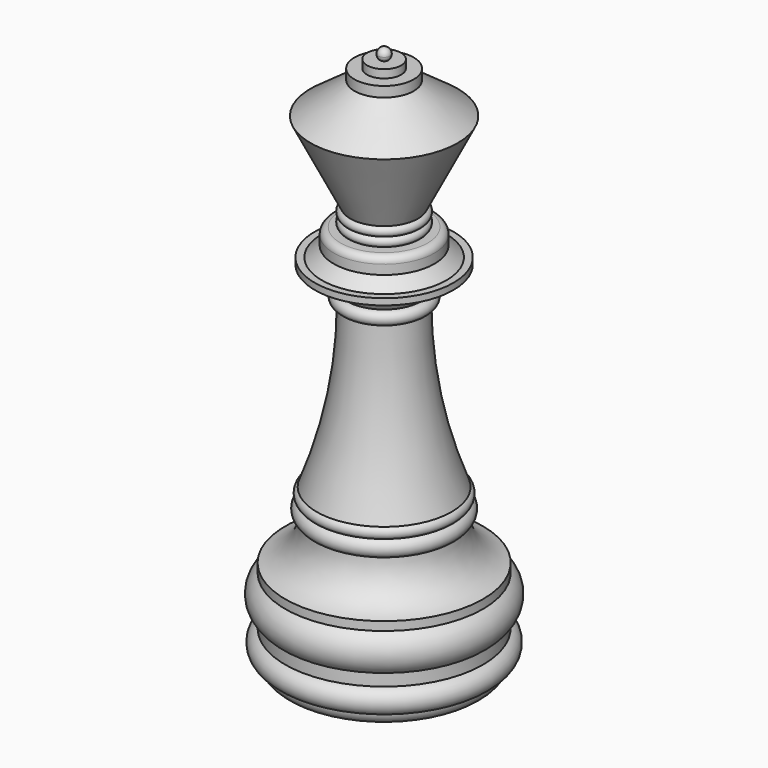
from build123d import *

# Parameters (mm, degrees)
F6_R     = 1
F8_R     = 0.896765
F9_DEPTH = 1.79353
F10_R    = 0.896755


# Not quite as in the source:
# - a fillet or chamfer that OpenCascade refuses, or shapes differently, is made with other operations: its cross-section is extruded or revolved along the edge and cut away or added
# - a fillet or chamfer is up to 0.001 mm smaller than in the source, because OpenCascade refuses the exact size


with BuildPart() as f1:
    # F0 (on Front) → F1 (revolve)
    with BuildSketch(Plane.XZ):
        with BuildLine():
            Line((-200.8288223515, 101.2477203459), (-203.3652514219, 101.2477203459))
            Line((-203.3652514219, 101.2477203459), (-203.3652514219, 21.2477203459))
            Line((-203.3652514219, 21.2477203459), (-188.6436624619, 21.2477203459))
            Line((-188.6436624619, 21.2477203459), (-188.6436624619, 23.0397097766))
            ThreePointArc((-188.6436624619, 23.0397097766), (-187.333962533, 24.8457370326), (-188.6436624619, 26.6517642885))
            Line((-188.6436624619, 26.6517642885), (-188.6436624619, 28.4437537193))
            ThreePointArc((-188.6436624619, 28.4437537193), (-187.1745849151, 31.1942528933), (-188.6436624619, 33.9447520673))
            Line((-188.6436624619, 33.9447520673), (-188.6436624619, 35.2401472628))
            Line((-188.6436624619, 35.2401472628), (-193.309366703, 35.2401472628))
            Line((-193.309366703, 35.2401472628), (-193.309366703, 41.1680191755))
            ThreePointArc((-193.309366703, 41.1680191755), (-192.5565818681, 42.3696450889), (-193.309366703, 43.5712710023))
            ThreePointArc((-193.309366703, 43.5712710023), (-192.8404048548, 44.3696901202), (-193.309366703, 45.1681092381))
            Line((-193.309366703, 45.1681092381), (-197.8608220816, 45.1681092381))
            Line((-197.8608220816, 45.1681092381), (-197.8608220816, 69.3112561437))
            ThreePointArc((-197.8608220816, 69.3112561437), (-196.8800943317, 70.2974423766), (-197.8608220816, 71.2836286096))
            Line((-197.8608220816, 71.2836286096), (-197.8608220816, 74.3284672499))
            Line((-197.8608220816, 74.3284672499), (-193.0439472198, 74.3284672499))
            Line((-193.0439472198, 74.3284672499), (-193.0439472198, 75.2748303938))
            Line((-193.0439472198, 75.2748303938), (-194.0847486258, 75.2748303938))
            Line((-194.0847486258, 75.2748303938), (-195.8655714989, 76.8517457771))
            Line((-195.8655714989, 76.8517457771), (-195.8655714989, 79.2579033303))
            Line((-195.8655714989, 79.2579033303), (-198.3242481947, 79.2579033303))
            ThreePointArc((-198.3242481947, 79.2579033303), (-197.7911045704, 79.9374569619), (-198.3242481947, 80.6170105934))
            ThreePointArc((-198.3242481947, 80.6170105934), (-197.7911045704, 81.296564225), (-198.3242481947, 81.9761178565))
            Line((-198.3242481947, 81.9761178565), (-192.4043744802, 93.8070736003))
            Line((-192.4043744802, 93.8070736003), (-198.949098587, 98.5011926961))
            Line((-198.949098587, 98.5011926961), (-198.949098587, 100.0268682092))
            Line((-198.949098587, 100.0268682092), (-200.8288223515, 100.0268682092))
            Line((-200.8288223515, 100.0268682092), (-200.8288223515, 101.2477203459))
        make_face()
    revolve(axis=Axis((-203.3652514219, 0, 61.2477203459), (0, 0, -1)))

    # F2: fillet of radius 2 on 1 edges, made by hand

    # F2_s1 → F2_t2 (revolve, cut)
    with BuildSketch(Plane.XZ):
        with BuildLine():
            ThreePointArc((-190.632815951, 21.2477203459), (-189.2941638562, 21.7617827398), (-188.6436624619, 23.0397097766))
            Line((-188.6436624619, 23.0397097766), (-188.6436624619, 21.2477203459))
            Line((-188.6436624619, 21.2477203459), (-190.632815951, 21.2477203459))
        make_face()
    revolve(axis=Axis((-203.3652514219, 0, 21.2477203459), (0, 0, -1)), mode=Mode.SUBTRACT)

    # F3: fillet of radius 6 on 1 edges, made by hand

    # F3_s1 → F3_t2 (revolve)
    with BuildSketch(Plane.XZ):
        with BuildLine():
            ThreePointArc((-193.309366703, 41.0899040806), (-192.0000902375, 37.3486325423), (-188.6436624619, 35.2401472628))
            Line((-188.6436624619, 35.2401472628), (-188.6703483771, 35.1231521265))
            ThreePointArc((-188.6703483771, 35.1231521265), (-190.9765145825, 35.1201472628), (-193.309366703, 35.1201472628))
            Line((-193.309366703, 35.1201472628), (-193.429366703, 35.2401472628))
            Line((-193.429366703, 35.2401472628), (-193.429366703, 41.0899040806))
            Line((-193.429366703, 41.0899040806), (-193.309366703, 41.0899040806))
        make_face()
    revolve(axis=Axis((-203.3652514219, 0, 35.2401472628), (0, 0, -1)))

    # F4: fillet of radius 66.3 on 1 edges, made by hand

    # F4_s1 → F4_t2 (revolve)
    with BuildSketch(Plane.XZ):
        with BuildLine():
            ThreePointArc((-197.8608220816, 69.3095101323), (-196.7130227674, 57.0261577479), (-193.309366703, 45.1681092381))
            Line((-193.309366703, 45.1681092381), (-194.5443375955, 44.6852812203))
            ThreePointArc((-194.5443375955, 44.6852812203), (-195.5850943923, 43.8421092381), (-197.8608220816, 43.8421092381))
            Line((-197.8608220816, 43.8421092381), (-199.1868220816, 45.1681092381))
            Line((-199.1868220816, 45.1681092381), (-199.1868220816, 69.3095101323))
            Line((-199.1868220816, 69.3095101323), (-197.8608220816, 69.3095101323))
        make_face()
    revolve(axis=Axis((-203.3652514219, 0, 45.1681092381), (0, 0, -1)))

    # F5: fillet of radius 5.33 on 1 edges, made by hand

    # F5_s1 → F5_t2 (revolve)
    with BuildSketch(Plane.XZ):
        with BuildLine():
            ThreePointArc((-193.0455404117, 74.3284672499), (-195.8941356754, 73.5033984395), (-197.8608220816, 71.2836286096))
            Line((-197.8608220816, 71.2836286096), (-197.957127715, 71.3293318368))
            ThreePointArc((-197.957127715, 71.3293318368), (-197.9674220816, 72.8060479297), (-197.9674220816, 74.3284672499))
            Line((-197.9674220816, 74.3284672499), (-197.8608220816, 74.4350672499))
            Line((-197.8608220816, 74.4350672499), (-193.0455404117, 74.4350672499))
            Line((-193.0455404117, 74.4350672499), (-193.0455404117, 74.3284672499))
        make_face()
    revolve(axis=Axis((-203.3652514219, 0, 74.3284672499), (0, 0, -1)))

    # F6
    f6_edges = [f1.edges().sort_by_distance(p)[0] for p in [
        (-210.864931, 0, 79.257903),
    ]]
    fillet(f6_edges, radius=F6_R)


with BuildPart() as f9:
    # F8 (on offset) → F9 (new body)
    with BuildSketch(Plane.XY.offset(101.0477203459)):
        with Locations((-203.3652514219, 0)):
            Circle(F8_R)
    extrude(amount=F9_DEPTH)

    # F10 (radius 0.896765 in the source; OpenCascade refuses exactly that, so slightly less here)
    f10_edges = [f9.edges().sort_by_distance(p)[0] for p in [
        (-204.262016, 0, 102.84125),
        (-204.262016, 0, 101.04772),
    ]]
    fillet(f10_edges, radius=F10_R)


solid = Compound([f1.part, f9.part])
